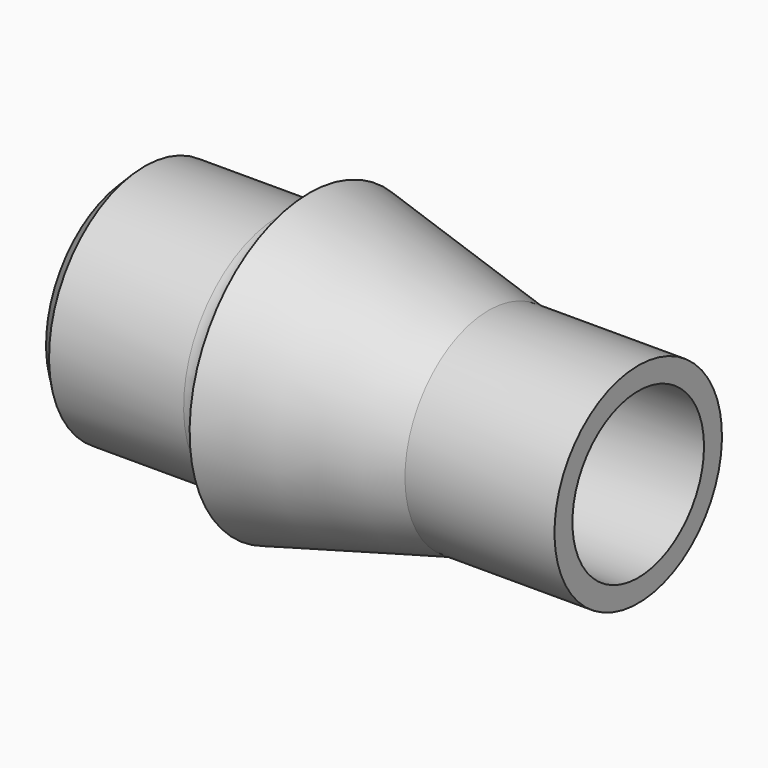
from build123d import *

# Parameters (mm, degrees)
F2_R     = 0.99999
F3_R     = 2.75
F4_DEPTH = 7.5
F5_R     = 1.75
F6_DEPTH = 9.5
F7_SIZE  = 0.5


# Not quite as in the source:
# - a fillet or chamfer is up to 0.001 mm smaller than in the source, because OpenCascade refuses the exact size


with BuildPart() as f1:
    # F0 (on Front) → F1 (revolve)
    with BuildSketch(Plane.XZ):
        Polygon((0, 4), (0, 0), (17, 0), (17, 3.5), (12, 3.5), (6, 5), (6, 4), align=None)
    revolve(axis=Axis((8.5, 0, 0), (-1, 0, 0)))

    # F2 (radius 1 in the source; OpenCascade refuses exactly that, so slightly less here)
    f2_edges = [f1.edges().sort_by_distance(p)[0] for p in [
        (6, 0, -4),
    ]]
    fillet(f2_edges, radius=F2_R)

    # F3 (on face) → F4 (cut)
    with BuildSketch(Plane.YZ.offset(17)):
        Circle(F3_R)
    extrude(amount=-F4_DEPTH, mode=Mode.SUBTRACT)

    # F5 (on face) → F6 (cut, through all)
    with BuildSketch(Plane(origin=(0, 0, 0), x_dir=(0, -1, 0), z_dir=(-1, 0, 0))):
        Circle(F5_R)
    extrude(amount=-F6_DEPTH, mode=Mode.SUBTRACT)

    # F7
    f7_edges = [f1.edges().sort_by_distance(p)[0] for p in [
        (0, 0, -4),
        (0, 1.75, 0),
    ]]
    chamfer(f7_edges, length=F7_SIZE)


solid = f1.part
